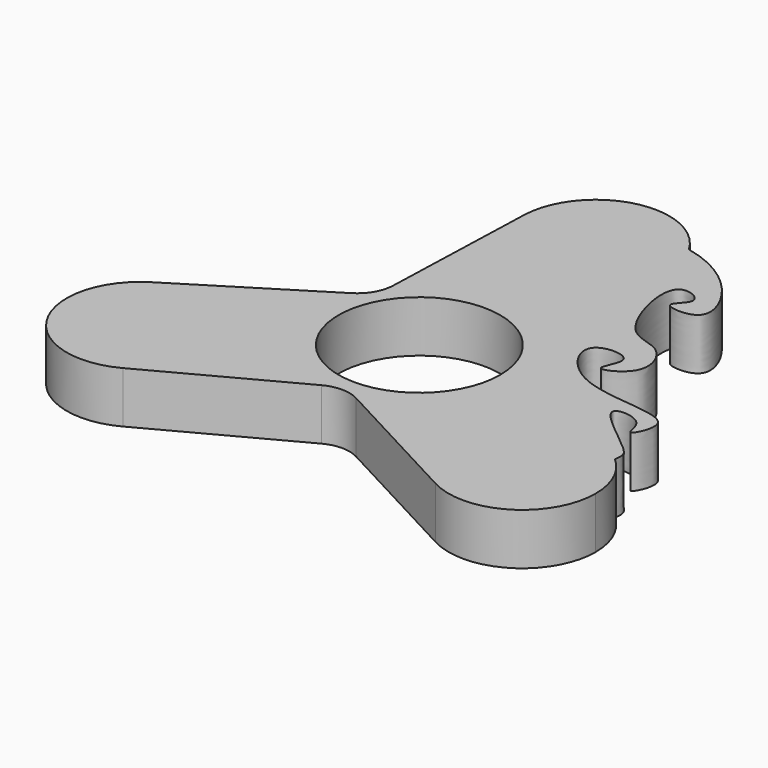
from build123d import *

# Parameters (mm, degrees)
F0_R     = 11
F1_DEPTH = 7


# Not quite as in the source:
# - a feature names something its author has since deleted; it is built from what else it names


with BuildPart() as f1:
    # F0 (on Top) → F1 (new body)
    with BuildSketch(Plane.XY):
        with BuildLine():
            ThreePointArc((-9.9944429004, 30.3333333333), (-0.1666898261, 20.0013893714), (10, 30))
            ThreePointArc((10, 30), (9.9986106286, 30.1666898261), (9.9944429004, 30.3333333333))
            ThreePointArc((9.9944429004, 30.3333333333), (9.6090466084, 32.7687945531), (8.6394201237, 35.0359130181))
            ThreePointArc((8.6394201237, 35.0359130181), (-2.4469543527, 39.6959999173), (-9.9944429004, 30.3333333333))
        make_face()
        with BuildLine():
            ThreePointArc((9.9944429004, 30.3333333333), (9.9986106286, 30.1666898261), (10, 30))
            ThreePointArc((10, 30), (-0.1666898261, 20.0013893714), (-9.9944429004, 30.3333333333))
            Line((-9.9944429004, 30.3333333333), (-10.7092358725, 8.9014606966))
            ThreePointArc((-10.7092358725, 8.9014606966), (-11.3763303038, 6.5681273633), (-13.0635090303, 4.8237399724))
            Line((-13.0635090303, 4.8237399724), (-31.2666586983, -6.5112252183))
            ThreePointArc((-31.2666586983, -6.5112252183), (-21.1258144232, -6.2576042801), (-15.9807621135, -15))
            ThreePointArc((-15.9807621135, -15), (-17.4050562197, -20.1436629382), (-21.2722157979, -23.8221081151))
            Line((-21.2722157979, -23.8221081151), (-2.3542731578, -13.725200669))
            ThreePointArc((-2.3542731578, -13.725200669), (0, -13.1362547266), (2.3542731578, -13.725200669))
            Line((2.3542731578, -13.725200669), (21.2722157979, -23.8221081151))
            ThreePointArc((21.2722157979, -23.8221081151), (17.3205080757, -10), (31.2666586983, -6.5112252183))
            Line((31.2666586983, -6.5112252183), (13.0635090303, 4.8237399724))
            ThreePointArc((13.0635090303, 4.8237399724), (11.3763303038, 6.5681273633), (10.7092358725, 8.9014606966))
            Line((10.7092358725, 8.9014606966), (9.9944429004, 30.3333333333))
        make_face()
        Circle(F0_R, mode=Mode.SUBTRACT)
        with BuildLine():
            ThreePointArc((8.6394201237, 35.0359130181), (9.6090466084, 32.7687945531), (9.9944429004, 30.3333333333))
            Line((9.9944429004, 30.3333333333), (10.7092358725, 8.9014606966))
            ThreePointArc((10.7092358725, 8.9014606966), (11.3763303038, 6.5681273633), (13.0635090303, 4.8237399724))
            Line((13.0635090303, 4.8237399724), (31.2666586983, -6.5112252183))
            ThreePointArc((31.2666586983, -6.5112252183), (31.9673374552, -6.9899490839), (32.6249052512, -7.5263555098))
            add(Edge.make_bspline(
                [(8.6394201237, 35.0359130181), (13.9791405245, 33.9313022187), (19.3345604365, 28.4670356067), (19.7766282836, 22.9262849119), (13.203703788, 23.3890528516), (17.9787416524, 26.3304847895), (11.0153121305, 29.3518202799), (14.6484703321, 15.1223253788), (20.567425968, 16.1514189079), (23.4237352348, 9.6032691823), (16.6512822907, 6.5366339201), (20.9070192695, 11.9751211188), (12.0944343738, 12.1881164979), (18.1879248471, 1.9951119769), (33.5912305893, 4.508093074), (29.6172838681, -3.4321747922), (30.0360748201, 1.4261029066), (22.1175057769, 1.8922728608), (33.001628255, -5.3665637563), (32.7576051866, -6.5185471211), (32.6249052512, -7.5263555098)],
                knots=[0, 0, 0, 0, 0.0885305165, 0.1362570633, 0.1827420963, 0.2230793888, 0.2658963137, 0.3449937205, 0.4015643726, 0.4579974818, 0.5065235559, 0.5502159866, 0.6007605945, 0.6688077756, 0.7563580334, 0.8027522302, 0.8416876616, 0.8880166736, 0.9621998701, 1, 1, 1, 1], degree=3))
        make_face()
        with BuildLine():
            ThreePointArc((35.9807621135, -15), (35.1033009974, -10.9037475283), (32.6249052512, -7.5263555098))
            ThreePointArc((32.6249052512, -7.5263555098), (31.9673374552, -6.9899490839), (31.2666586983, -6.5112252183))
            ThreePointArc((31.2666586983, -6.5112252183), (17.3205080757, -10), (21.2722157979, -23.8221081151))
            ThreePointArc((21.2722157979, -23.8221081151), (31.1244250518, -23.5757058939), (35.9807621135, -15))
        make_face()
        with BuildLine():
            ThreePointArc((-15.9807621135, -15), (-21.1258144232, -6.2576042801), (-31.2666586983, -6.5112252183))
            ThreePointArc((-31.2666586983, -6.5112252183), (-34.6410161514, -20), (-21.2722157979, -23.8221081151))
            ThreePointArc((-21.2722157979, -23.8221081151), (-17.4050562197, -20.1436629382), (-15.9807621135, -15))
        make_face()
    extrude(amount=F1_DEPTH)


solid = f1.part
